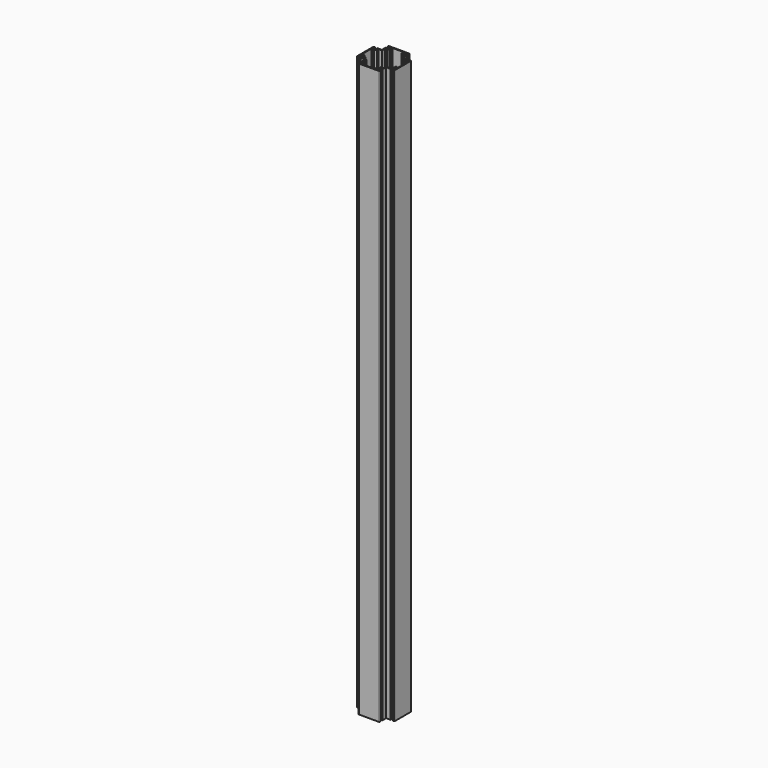
from build123d import *

# Parameters (mm, degrees)
F1_DEPTH = 2726
F2_T     = -4
F3_R     = 3
F4_W     = 3
F4_H     = 4
F4_W_2   = 4
F4_H_2   = 11
F4_W_3   = 11
F4_H_3   = 3
F5_DEPTH = 2726


# Not quite as in the source:
# - a shell that OpenCascade refuses in one call is made with other operations: the cavity is built on its own and cut out


with BuildPart() as f1:
    # F0 (on Top) → F1 (new body)
    with BuildSketch(Plane.XY):
        Polygon((50, 90), (-50, 90), (-50, 82), (-46, 82), (-46, 86), (-38, 86), (-38, 68), (-46, 68), (-46, 72), (-50, 72), (-50, 50), (-72, 50), (-72, 46), (-68, 46), (-68, 38), (-86, 38), (-86, 46), (-82, 46), (-82, 50), (-90, 50), (-90, -50), (-82, -50), (-82, -46), (-86, -46), (-86, -38), (-68, -38), (-68, -46), (-72, -46), (-72, -50), (-50, -50), (-50, -72), (-46, -72), (-46, -68), (-38, -68), (-38, -86), (-46, -86), (-46, -82), (-50, -82), (-50, -90), (50, -90), (50, -82), (46, -82), (46, -86), (38, -86), (38, -68), (46, -68), (46, -72), (50, -72), (50, -50), (72, -50), (72, -46), (68, -46), (68, -38), (86, -38), (86, -46), (82, -46), (82, -50), (90, -50), (90, 50), (82, 50), (82, 46), (86, 46), (86, 38), (68, 38), (68, 46), (72, 46), (72, 50), (50, 50), (50, 72), (46, 72), (46, 68), (38, 68), (38, 86), (46, 86), (46, 82), (50, 82), align=None)
    extrude(amount=F1_DEPTH)

    # F2: a shell. OpenCascade refuses it in one call, so the cavity is built on its own and cut out:
    # the body offset inwards by the wall thickness, plus a prism from it out through each open face.
    f2_core = offset(f1.part, amount=F2_T, kind=Kind.INTERSECTION, mode=Mode.PRIVATE)
    f2_exits = [f2_core.faces().sort_by_distance(p)[0] for p in [
        (0, 0, 2722),
        (0, 0, 4),
    ]]
    add(f2_core, mode=Mode.SUBTRACT)
    extrude(f2_exits, amount=-F2_T, mode=Mode.SUBTRACT)

    # F3
    f3_edges = [f1.edges().sort_by_distance(p)[0] for p in [
        (-50, -90, 1363),
        (-90, -50, 1363),
        (50, -90, 1363),
        (90, -50, 1363),
        (90, 50, 1363),
        (50, 90, 1363),
        (-50, 90, 1363),
        (-90, 50, 1363),
    ]]
    fillet(f3_edges, radius=F3_R)

    # F4 (on face) → F5 (join, through all)
    with BuildSketch(Plane(origin=(0, 0, 0), x_dir=(1, 0, 0), z_dir=(0, 0, -1))):
        with Locations((-62.5, 36)):
            Rectangle(F4_W, F4_H)
        with Locations((-76, 28.5)):
            Rectangle(F4_W_2, F4_H_2)
        with Locations((62.5, 36)):
            Rectangle(F4_W, F4_H)
        with Locations((76, 28.5)):
            Rectangle(F4_W_2, F4_H_2)
        with Locations((76, -28.5)):
            Rectangle(F4_W_2, F4_H_2)
        with Locations((62.5, -36)):
            Rectangle(F4_W, F4_H)
        with Locations((-62.5, -36)):
            Rectangle(F4_W, F4_H)
        with Locations((-76, -28.5)):
            Rectangle(F4_W_2, F4_H_2)
        with Locations((-28.5, 76)):
            Rectangle(F4_W_3, F4_H)
        with Locations((-36, 62.5)):
            Rectangle(F4_W_2, F4_H_3)
        with Locations((28.5, 76)):
            Rectangle(F4_W_3, F4_H)
        with Locations((36, 62.5)):
            Rectangle(F4_W_2, F4_H_3)
        with Locations((-28.5, -76)):
            Rectangle(F4_W_3, F4_H)
        with Locations((36, -62.5)):
            Rectangle(F4_W_2, F4_H_3)
        with Locations((-36, -62.5)):
            Rectangle(F4_W_2, F4_H_3)
        with Locations((28.5, -76)):
            Rectangle(F4_W_3, F4_H)
    extrude(amount=-F5_DEPTH)


solid = f1.part
